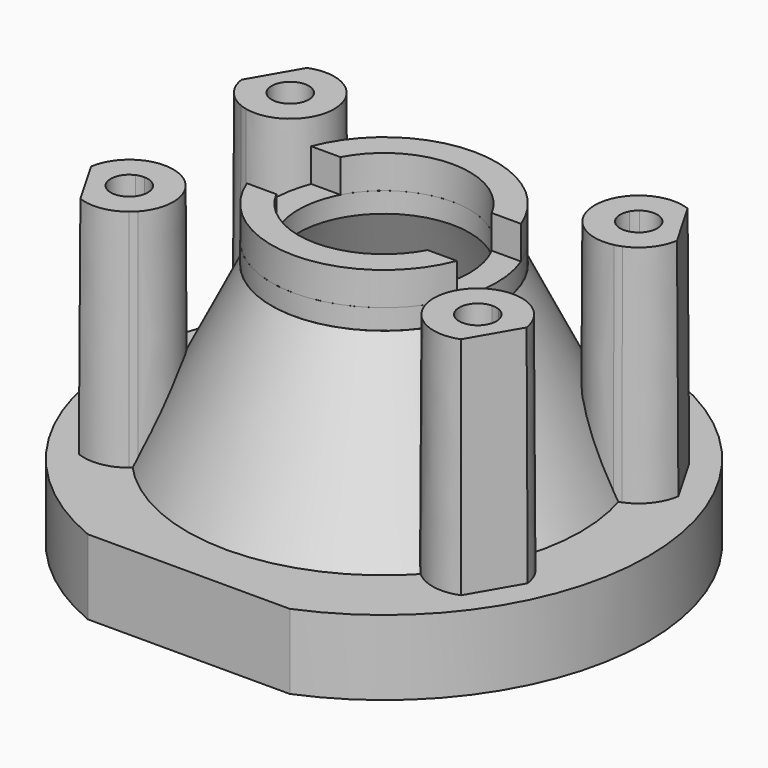
from build123d import *

# Parameters (mm, degrees)
F0_R                     = 9.144
F1_DEPTH                 = 3.556
F3_DEPTH                 = 10.668
DRAFT_F3_DRAFTED_ANGLE   = 0.3
DRAFT_F3_2_DRAFTED_ANGLE = 0.3
DRAFT_F3_3_DRAFTED_ANGLE = 0.3
DRAFT_F3_4_DRAFTED_ANGLE = 0.3
F5_DEPTH                 = 1.5748
F6_R                     = 5.334
F6_R_2                   = 4.064
F7_DEPTH                 = 0.9652


# Not quite as in the source:
# - an extrude with a draft is written as a straight extrude whose walls are then drafted


with BuildPart() as f1:
    # F0 (on Top) → F1 (new body)
    with BuildSketch(Plane.XY):
        with BuildLine():
            Line((4.7928830833, 11.5824), (-4.7928830833, 11.5824))
            ThreePointArc((-4.7928830833, 11.5824), (-12.5349, 0), (-4.7928830833, -11.5824))
            Line((-4.7928830833, -11.5824), (4.7928830833, -11.5824))
            ThreePointArc((4.7928830833, -11.5824), (12.5349, 0), (4.7928830833, 11.5824))
        make_face()
        Circle(F0_R, mode=Mode.SUBTRACT)
    extrude(amount=F1_DEPTH)


with BuildPart() as f3_drafted:
    # F2 (on face) → F3 (new body)
    with BuildSketch(Plane.XY.offset(3.556)):
        with BuildLine():
            ThreePointArc((8.7420594313, 2.6812558436), (8.9078225485, 2.7255855568), (9.0695147841, 2.7830151258))
            ThreePointArc((9.0695147841, 2.7830151258), (8.8537236445, 3.4077630841), (8.5949555805, 4.0159693947))
            ThreePointArc((8.5949555805, 4.0159693947), (8.4244599224, 3.9641104693), (8.2468072886, 3.9500513344))
            ThreePointArc((8.2468072886, 3.9500513344), (8.5180900797, 3.3248875761), (8.7420594313, 2.6812558436))
        make_face()
        with BuildLine():
            ThreePointArc((8.5949555805, 4.0159693947), (8.8537236445, 3.4077630841), (9.0695147841, 2.7830151258))
            ThreePointArc((9.0695147841, 2.7830151258), (9.9593005644, 3.4501074997), (10.395799934, 4.4729463289))
            Line((10.395799934, 4.4729463289), (9.0715851176, 6.7665536711))
            ThreePointArc((9.0715851176, 6.7665536711), (7.9675310228, 6.8999535428), (6.9449191901, 6.4629226402))
            ThreePointArc((6.9449191901, 6.4629226402), (7.3780712231, 5.9636680522), (7.7754093069, 5.4354651797))
            ThreePointArc((7.7754093069, 5.4354651797), (8.6399633651, 5.5135998748), (9.0963890163, 4.7752))
            ThreePointArc((9.0963890163, 4.7752), (8.9597167156, 4.3202641247), (8.5949555805, 4.0159693947))
        make_face()
        with BuildLine():
            ThreePointArc((6.6930653903, 6.2302176271), (6.4121386922, 3.70205), (8.7420594313, 2.6812558436))
            ThreePointArc((8.7420594313, 2.6812558436), (8.5180900797, 3.3248875761), (8.2468072886, 3.9500513344))
            ThreePointArc((8.2468072886, 3.9500513344), (7.5559850455, 4.36245), (7.5442484461, 5.1669189449))
            ThreePointArc((7.5442484461, 5.1669189449), (7.1384821455, 5.7144386127), (6.6930653903, 6.2302176271))
        make_face()
        with BuildLine():
            ThreePointArc((7.5442484461, 5.1669189449), (7.645250331, 5.3137410713), (7.7754093069, 5.4354651797))
            ThreePointArc((7.7754093069, 5.4354651797), (7.3780712231, 5.9636680522), (6.9449191901, 6.4629226402))
            ThreePointArc((6.9449191901, 6.4629226402), (6.8143376066, 6.3516078409), (6.6930653903, 6.2302176271))
            ThreePointArc((6.6930653903, 6.2302176271), (7.1384821455, 5.7144386127), (7.5442484461, 5.1669189449))
        make_face()
    extrude(amount=F3_DEPTH)

    # draft_F3_drafted
    draft_f3_drafted_walls = [f3_drafted.faces().sort_by_distance(p)[0] for p in [
        (9.7336925258, 5.61975, 10.668),
        (6.4121386922, 3.70205, 10.668),
        (8.9975295865, 4.3834810551, 10.668),
    ]]
    draft(draft_f3_drafted_walls, neutral_plane=Plane.XY.offset(3.556), angle=DRAFT_F3_DRAFTED_ANGLE)


with BuildPart() as f1_1:
    add(f1.part)

    # join_F3_drafted: union F3_drafted
    add(f3_drafted.part)


with BuildPart() as f3_2_drafted:
    # F2 (on face) → F3, piece 2 (new body)
    with BuildSketch(Plane.XY.offset(3.556)):
        with BuildLine():
            ThreePointArc((10.395799934, -4.4729463289), (9.9593005644, -3.4501074997), (9.0695147841, -2.7830151258))
            ThreePointArc((9.0695147841, -2.7830151258), (8.8537236445, -3.4077630841), (8.5949555805, -4.0159693947))
            ThreePointArc((8.5949555805, -4.0159693947), (8.9597167156, -4.3202641247), (9.0963890163, -4.7752))
            ThreePointArc((9.0963890163, -4.7752), (8.6399633651, -5.5135998748), (7.7754093069, -5.4354651797))
            ThreePointArc((7.7754093069, -5.4354651797), (7.3780712231, -5.9636680522), (6.9449191901, -6.4629226402))
            ThreePointArc((6.9449191901, -6.4629226402), (7.9675310228, -6.8999535428), (9.0715851176, -6.7665536711))
            Line((9.0715851176, -6.7665536711), (10.395799934, -4.4729463289))
        make_face()
        with BuildLine():
            ThreePointArc((8.5949555805, -4.0159693947), (8.8537236445, -3.4077630841), (9.0695147841, -2.7830151258))
            ThreePointArc((9.0695147841, -2.7830151258), (8.9078225485, -2.7255855568), (8.7420594313, -2.6812558436))
            ThreePointArc((8.7420594313, -2.6812558436), (8.5180900797, -3.3248875761), (8.2468072886, -3.9500513344))
            ThreePointArc((8.2468072886, -3.9500513344), (8.4244599224, -3.9641104693), (8.5949555805, -4.0159693947))
        make_face()
        with BuildLine():
            ThreePointArc((8.2468072886, -3.9500513344), (8.5180900797, -3.3248875761), (8.7420594313, -2.6812558436))
            ThreePointArc((8.7420594313, -2.6812558436), (6.4121386922, -3.70205), (6.6930653903, -6.2302176271))
            ThreePointArc((6.6930653903, -6.2302176271), (7.1384821455, -5.7144386127), (7.5442484461, -5.1669189449))
            ThreePointArc((7.5442484461, -5.1669189449), (7.5559850455, -4.36245), (8.2468072886, -3.9500513344))
        make_face()
        with BuildLine():
            ThreePointArc((6.9449191901, -6.4629226402), (7.3780712231, -5.9636680522), (7.7754093069, -5.4354651797))
            ThreePointArc((7.7754093069, -5.4354651797), (7.645250331, -5.3137410713), (7.5442484461, -5.1669189449))
            ThreePointArc((7.5442484461, -5.1669189449), (7.1384821455, -5.7144386127), (6.6930653903, -6.2302176271))
            ThreePointArc((6.6930653903, -6.2302176271), (6.8143376066, -6.3516078409), (6.9449191901, -6.4629226402))
        make_face()
    extrude(amount=F3_DEPTH)

    # draft_F3_2_drafted
    draft_f3_2_drafted_walls = [f3_2_drafted.faces().sort_by_distance(p)[0] for p in [
        (9.7336925258, -5.61975, 10.668),
        (6.4121386922, -3.70205, 10.668),
        (8.7663687257, -4.1149348203, 10.668),
    ]]
    draft(draft_f3_2_drafted_walls, neutral_plane=Plane.XY.offset(3.556), angle=DRAFT_F3_2_DRAFTED_ANGLE)


with BuildPart() as f1_2:
    add(f1_1.part)

    # join_F3_2_drafted: union F3_2_drafted
    add(f3_2_drafted.part)


with BuildPart() as f3_3_drafted:
    # F2 (on face) → F3, piece 3 (new body)
    with BuildSketch(Plane.XY.offset(3.556)):
        with BuildLine():
            ThreePointArc((-7.5442484461, 5.1669189449), (-7.1384821455, 5.7144386127), (-6.6930653903, 6.2302176271))
            ThreePointArc((-6.6930653903, 6.2302176271), (-6.8143376066, 6.3516078409), (-6.9449191901, 6.4629226402))
            ThreePointArc((-6.9449191901, 6.4629226402), (-7.3780712231, 5.9636680522), (-7.7754093069, 5.4354651797))
            ThreePointArc((-7.7754093069, 5.4354651797), (-7.645250331, 5.3137410713), (-7.5442484461, 5.1669189449))
        make_face()
        with BuildLine():
            ThreePointArc((-8.7420594313, 2.6812558436), (-6.4121386922, 3.70205), (-6.6930653903, 6.2302176271))
            ThreePointArc((-6.6930653903, 6.2302176271), (-7.1384821455, 5.7144386127), (-7.5442484461, 5.1669189449))
            ThreePointArc((-7.5442484461, 5.1669189449), (-7.4704853554, 4.9772005685), (-7.4453890163, 4.7752))
            ThreePointArc((-7.4453890163, 4.7752), (-7.6787193969, 4.2000605457), (-8.2468072886, 3.9500513344))
            ThreePointArc((-8.2468072886, 3.9500513344), (-8.5180900797, 3.3248875761), (-8.7420594313, 2.6812558436))
        make_face()
        with BuildLine():
            ThreePointArc((-7.7754093069, 5.4354651797), (-7.3780712231, 5.9636680522), (-6.9449191901, 6.4629226402))
            ThreePointArc((-6.9449191901, 6.4629226402), (-7.9675310228, 6.8999535428), (-9.0715851176, 6.7665536711))
            Line((-9.0715851176, 6.7665536711), (-10.395799934, 4.4729463289))
            ThreePointArc((-10.395799934, 4.4729463289), (-9.9593005644, 3.4501074997), (-9.0695147841, 2.7830151258))
            ThreePointArc((-9.0695147841, 2.7830151258), (-8.8537236445, 3.4077630841), (-8.5949555805, 4.0159693947))
            ThreePointArc((-8.5949555805, 4.0159693947), (-8.9857929871, 5.18795), (-7.7754093069, 5.4354651797))
        make_face()
        with BuildLine():
            ThreePointArc((-9.0695147841, 2.7830151258), (-8.9078225485, 2.7255855568), (-8.7420594313, 2.6812558436))
            ThreePointArc((-8.7420594313, 2.6812558436), (-8.5180900797, 3.3248875761), (-8.2468072886, 3.9500513344))
            ThreePointArc((-8.2468072886, 3.9500513344), (-8.4244599224, 3.9641104693), (-8.5949555805, 4.0159693947))
            ThreePointArc((-8.5949555805, 4.0159693947), (-8.8537236445, 3.4077630841), (-9.0695147841, 2.7830151258))
        make_face()
    extrude(amount=F3_DEPTH)

    # draft_F3_3_drafted
    draft_f3_3_drafted_walls = [f3_3_drafted.faces().sort_by_distance(p)[0] for p in [
        (-9.7336925258, 5.61975, 10.668),
        (-6.4121386922, 3.70205, 10.668),
        (-8.294970744, 5.6003486656, 10.668),
    ]]
    draft(draft_f3_3_drafted_walls, neutral_plane=Plane.XY.offset(3.556), angle=DRAFT_F3_3_DRAFTED_ANGLE)


with BuildPart() as f1_3:
    add(f1_2.part)

    # join_F3_3_drafted: union F3_3_drafted
    add(f3_3_drafted.part)


with BuildPart() as f3_4_drafted:
    # F2 (on face) → F3, piece 4 (new body)
    with BuildSketch(Plane.XY.offset(3.556)):
        with BuildLine():
            ThreePointArc((-7.5442484461, -5.1669189449), (-7.1384821455, -5.7144386127), (-6.6930653903, -6.2302176271))
            ThreePointArc((-6.6930653903, -6.2302176271), (-6.4121386922, -3.70205), (-8.7420594313, -2.6812558436))
            ThreePointArc((-8.7420594313, -2.6812558436), (-8.5180900797, -3.3248875761), (-8.2468072886, -3.9500513344))
            ThreePointArc((-8.2468072886, -3.9500513344), (-7.6787193969, -4.2000605457), (-7.4453890163, -4.7752))
            ThreePointArc((-7.4453890163, -4.7752), (-7.4704853554, -4.9772005685), (-7.5442484461, -5.1669189449))
        make_face()
        with BuildLine():
            ThreePointArc((-6.9449191901, -6.4629226402), (-6.8143376066, -6.3516078409), (-6.6930653903, -6.2302176271))
            ThreePointArc((-6.6930653903, -6.2302176271), (-7.1384821455, -5.7144386127), (-7.5442484461, -5.1669189449))
            ThreePointArc((-7.5442484461, -5.1669189449), (-7.645250331, -5.3137410713), (-7.7754093069, -5.4354651797))
            ThreePointArc((-7.7754093069, -5.4354651797), (-7.3780712231, -5.9636680522), (-6.9449191901, -6.4629226402))
        make_face()
        with BuildLine():
            ThreePointArc((-9.0715851176, -6.7665536711), (-7.9675310228, -6.8999535428), (-6.9449191901, -6.4629226402))
            ThreePointArc((-6.9449191901, -6.4629226402), (-7.3780712231, -5.9636680522), (-7.7754093069, -5.4354651797))
            ThreePointArc((-7.7754093069, -5.4354651797), (-8.9857929871, -5.18795), (-8.5949555805, -4.0159693947))
            ThreePointArc((-8.5949555805, -4.0159693947), (-8.8537236445, -3.4077630841), (-9.0695147841, -2.7830151258))
            ThreePointArc((-9.0695147841, -2.7830151258), (-9.9593005644, -3.4501074997), (-10.395799934, -4.4729463289))
            Line((-10.395799934, -4.4729463289), (-9.0715851176, -6.7665536711))
        make_face()
        with BuildLine():
            ThreePointArc((-8.2468072886, -3.9500513344), (-8.5180900797, -3.3248875761), (-8.7420594313, -2.6812558436))
            ThreePointArc((-8.7420594313, -2.6812558436), (-8.9078225485, -2.7255855568), (-9.0695147841, -2.7830151258))
            ThreePointArc((-9.0695147841, -2.7830151258), (-8.8537236445, -3.4077630841), (-8.5949555805, -4.0159693947))
            ThreePointArc((-8.5949555805, -4.0159693947), (-8.4244599224, -3.9641104693), (-8.2468072886, -3.9500513344))
        make_face()
    extrude(amount=F3_DEPTH)

    # draft_F3_4_drafted
    draft_f3_4_drafted_walls = [f3_4_drafted.faces().sort_by_distance(p)[0] for p in [
        (-7.9468224521, -5.5344306053, 10.668),
        (-9.7336925258, -5.61975, 10.668),
        (-6.4121386922, -3.70205, 10.668),
    ]]
    draft(draft_f3_4_drafted_walls, neutral_plane=Plane.XY.offset(3.556), angle=DRAFT_F3_4_DRAFTED_ANGLE)


with BuildPart() as f1_4:
    add(f1_3.part)

    # join_F3_4_drafted: union F3_4_drafted
    add(f3_4_drafted.part)


with BuildPart() as f5:
    # F4 (on face) → F5 (new body)
    with BuildSketch(Plane.XY.offset(14.224)):
        with BuildLine():
            Line((-3.5898566824, -1.905), (-4.9822214925, -1.905))
            ThreePointArc((-4.9822214925, -1.905), (0, -5.334), (4.9822214925, -1.905))
            Line((4.9822214925, -1.905), (3.5898566824, -1.905))
            ThreePointArc((3.5898566824, -1.905), (0, -4.064), (-3.5898566824, -1.905))
        make_face()
    extrude(amount=-F5_DEPTH)


with BuildPart() as f5b:
    # F4 (on face) → F5, piece 2 (new body)
    with BuildSketch(Plane.XY.offset(14.224)):
        with BuildLine():
            ThreePointArc((-3.5898566824, 1.905), (0, 4.064), (3.5898566824, 1.905))
            Line((3.5898566824, 1.905), (4.9822214925, 1.905))
            ThreePointArc((4.9822214925, 1.905), (0, 5.334), (-4.9822214925, 1.905))
            Line((-4.9822214925, 1.905), (-3.5898566824, 1.905))
        make_face()
    extrude(amount=-F5_DEPTH)


with BuildPart() as f7:
    # F6 (on face) → F7 (new body)
    with BuildSketch(Plane(origin=(0, 0, 12.6492), x_dir=(1, 0, 0), z_dir=(0, 0, -1))):
        Circle(F6_R)
        Circle(F6_R_2, mode=Mode.SUBTRACT)
    extrude(amount=F7_DEPTH)


with BuildPart() as f9:
    # F8 (on Right) → F9 (revolve)
    with BuildSketch(Plane.YZ):
        Polygon((9.3497093767, 3.556), (5.3382301703, 11.684), (4.7413497232, 11.684), (8.7545045163, 3.5526049508), align=None)
    revolve(axis=Axis((0, 0, 1.8133264966), (0, 0, 1)))


solid = Compound([f1_4.part, f5.part, f5b.part, f7.part, f9.part])
